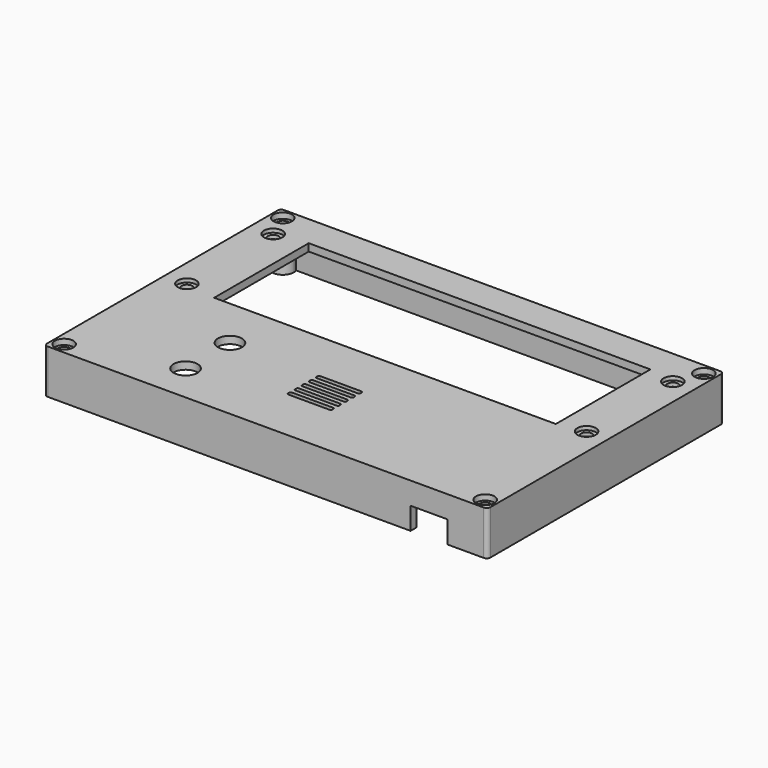
from build123d import *

# Parameters (mm, degrees)
F0_W            = 120
F0_H            = 80
F1_DEPTH        = 2
F3_DEPTH        = 12
F5_D            = 3
F5_CBORE_D      = 5
F5_CBORE_DEPTH  = 1
F4_W            = 92.5
F4_H            = 32
F6_DEPTH        = 3
F7_W            = 10
F7_H            = 6
F8_DEPTH        = 3
F9_R            = 1
F10_R           = 3.25
F11_DEPTH       = 2
F12_R           = 1.25
F13_DEPTH       = 1
F15_D           = 3.2
F15_CBORE_D     = 5
F15_CBORE_DEPTH = 1.5


# Not quite as in the source:
# - a feature names something its author has since deleted; it is built from what else it names


with BuildPart() as f1:
    # F0 (on Top) → F1 (new body)
    with BuildSketch(Plane.XY):
        Rectangle(F0_W, F0_H)
    extrude(amount=F1_DEPTH)

    # F2 (on face) → F3 (join)
    with BuildSketch(Plane.XY.offset(2)):
        with BuildLine():
            Line((-58, 38), (-54.1715728753, 38))
            ThreePointArc((-54.1715728753, 38), (-55.2679491924, 39.4494897428), (-57, 40))
            ThreePointArc((-57, 40), (-59.1213203436, 39.1213203436), (-60, 37))
            ThreePointArc((-60, 37), (-59.4494897428, 35.2679491924), (-58, 34.1715728753))
            Line((-58, 34.1715728753), (-58, 38))
        make_face()
        with BuildLine():
            ThreePointArc((-60, 37), (-59.1213203436, 39.1213203436), (-57, 40))
            Line((-57, 40), (-60, 40))
            Line((-60, 40), (-60, 37))
        make_face()
        with BuildLine():
            ThreePointArc((-54, 37), (-54.043204321, 37.5073059362), (-54.1715728753, 38))
            Line((-54.1715728753, 38), (-58, 38))
            Line((-58, 38), (-58, 34.1715728753))
            ThreePointArc((-58, 34.1715728753), (-55.2679491924, 34.5505102572), (-54, 37))
        make_face()
        with BuildLine():
            Line((-58, -34.1715728753), (-58, 34.1715728753))
            ThreePointArc((-58, 34.1715728753), (-59.4494897428, 35.2679491924), (-60, 37))
            Line((-60, 37), (-60, -37))
            ThreePointArc((-60, -37), (-59.4494897428, -35.2679491924), (-58, -34.1715728753))
        make_face()
        with BuildLine():
            Line((-54.1715728753, 38), (54.1715728753, 38))
            ThreePointArc((54.1715728753, 38), (55.2679491924, 39.4494897428), (57, 40))
            Line((57, 40), (-57, 40))
            ThreePointArc((-57, 40), (-55.2679491924, 39.4494897428), (-54.1715728753, 38))
        make_face()
        with BuildLine():
            Line((54.1715728753, 38), (58, 38))
            Line((58, 38), (58, 34.1715728753))
            ThreePointArc((58, 34.1715728753), (59.4494897428, 35.2679491924), (60, 37))
            ThreePointArc((60, 37), (59.1213203436, 39.1213203436), (57, 40))
            ThreePointArc((57, 40), (55.2679491924, 39.4494897428), (54.1715728753, 38))
        make_face()
        with BuildLine():
            Line((58, 34.1715728753), (58, 38))
            Line((58, 38), (54.1715728753, 38))
            ThreePointArc((54.1715728753, 38), (54.8786796564, 34.8786796564), (58, 34.1715728753))
        make_face()
        with BuildLine():
            Line((60, 40), (57, 40))
            ThreePointArc((57, 40), (59.1213203436, 39.1213203436), (60, 37))
            Line((60, 37), (60, 40))
        make_face()
        with BuildLine():
            ThreePointArc((60, 37), (59.4494897428, 35.2679491924), (58, 34.1715728753))
            Line((58, 34.1715728753), (58, -34.1715728753))
            ThreePointArc((58, -34.1715728753), (59.4494897428, -35.2679491924), (60, -37))
            Line((60, -37), (60, 37))
        make_face()
        with BuildLine():
            Line((60, -40), (60, -37))
            ThreePointArc((60, -37), (59.1213203436, -39.1213203436), (57, -40))
            Line((57, -40), (60, -40))
        make_face()
        with BuildLine():
            ThreePointArc((60, -37), (59.4494897428, -35.2679491924), (58, -34.1715728753))
            Line((58, -34.1715728753), (58, -38))
            Line((58, -38), (54.1715728753, -38))
            ThreePointArc((54.1715728753, -38), (55.2679491924, -39.4494897428), (57, -40))
            ThreePointArc((57, -40), (59.1213203436, -39.1213203436), (60, -37))
        make_face()
        with BuildLine():
            Line((58, -38), (58, -34.1715728753))
            ThreePointArc((58, -34.1715728753), (54.8786796564, -34.8786796564), (54.1715728753, -38))
            Line((54.1715728753, -38), (58, -38))
        make_face()
        with BuildLine():
            ThreePointArc((57, -40), (55.2679491924, -39.4494897428), (54.1715728753, -38))
            Line((54.1715728753, -38), (-54.1715728753, -38))
            ThreePointArc((-54.1715728753, -38), (-55.2679491924, -39.4494897428), (-57, -40))
            Line((-57, -40), (57, -40))
        make_face()
        with BuildLine():
            ThreePointArc((-57, -40), (-59.1213203436, -39.1213203436), (-60, -37))
            Line((-60, -37), (-60, -40))
            Line((-60, -40), (-57, -40))
        make_face()
        with BuildLine():
            ThreePointArc((-57, -40), (-55.2679491924, -39.4494897428), (-54.1715728753, -38))
            Line((-54.1715728753, -38), (-58, -38))
            Line((-58, -38), (-58, -34.1715728753))
            ThreePointArc((-58, -34.1715728753), (-59.4494897428, -35.2679491924), (-60, -37))
            ThreePointArc((-60, -37), (-59.1213203436, -39.1213203436), (-57, -40))
        make_face()
        with BuildLine():
            Line((-58, -38), (-54.1715728753, -38))
            ThreePointArc((-54.1715728753, -38), (-54.043204321, -37.5073059362), (-54, -37))
            ThreePointArc((-54, -37), (-55.2679491924, -34.5505102572), (-58, -34.1715728753))
            Line((-58, -34.1715728753), (-58, -38))
        make_face()
    extrude(amount=-F3_DEPTH)

    # F5 (through all)
    with Locations(Plane.XY.offset(2)):
        with Locations((-54, 30), (-54, 0.8), (54.2, 0.8), (54.2, 30)):
            CounterBoreHole(F5_D / 2, F5_CBORE_D / 2, F5_CBORE_DEPTH)

    # F4 (on face) → F6 (cut)
    with BuildSketch(Plane.XY.offset(2)):
        with Locations((0.75, 15.4)):
            Rectangle(F4_W, F4_H)
    extrude(amount=-F6_DEPTH, mode=Mode.SUBTRACT)

    # F7 (on face) → F8 (cut)
    with BuildSketch(Plane.XZ.offset(40)):
        with Locations((44.2, -7)):
            Rectangle(F7_W, F7_H)
    extrude(amount=-F8_DEPTH, mode=Mode.SUBTRACT)

    # F9
    f9_edges = [f1.edges().sort_by_distance(p)[0] for p in [
        (60, -40, -4),
        (60, 40, -4),
        (-60, -40, -4),
        (-60, 40, -4),
    ]]
    fillet(f9_edges, radius=F9_R)

    # F10 (on face) → F11 (cut, through all)
    with BuildSketch(Plane.XY.offset(2)):
        with Locations((-30, -14.6378241479)):
            Circle(F10_R)
        with Locations((-30, -29.6378241479)):
            Circle(F10_R)
        with BuildLine():
            Line((-5.6, -15.8000669783), (5.6, -15.8000669783))
            ThreePointArc((5.6, -15.8000669783), (5.8828427125, -15.6829096908), (6, -15.4000669783))
            Line((6, -15.4000669783), (6, -15.0000669783))
            ThreePointArc((6, -15.0000669783), (5.8828427125, -14.7172242658), (5.6, -14.6000669783))
            Line((5.6, -14.6000669783), (-5.6, -14.6000669783))
            ThreePointArc((-5.6, -14.6000669783), (-5.8828427125, -14.7172242658), (-6, -15.0000669783))
            Line((-6, -15.0000669783), (-6, -15.4000669783))
            ThreePointArc((-6, -15.4000669783), (-5.8828427125, -15.6829096908), (-5.6, -15.8000669783))
        make_face()
        with BuildLine():
            ThreePointArc((6, -17.4000669783), (5.8828427125, -17.1172242658), (5.6, -17.0000669783))
            Line((5.6, -17.0000669783), (-5.6, -17.0000669783))
            ThreePointArc((-5.6, -17.0000669783), (-5.8828427125, -17.1172242658), (-6, -17.4000669783))
            Line((-6, -17.4000669783), (-6, -17.8000669783))
            ThreePointArc((-6, -17.8000669783), (-5.8828427125, -18.0829096908), (-5.6, -18.2000669783))
            Line((-5.6, -18.2000669783), (5.6, -18.2000669783))
            ThreePointArc((5.6, -18.2000669783), (5.8828427125, -18.0829096908), (6, -17.8000669783))
            Line((6, -17.8000669783), (6, -17.4000669783))
        make_face()
        with BuildLine():
            ThreePointArc((6, -19.8000669783), (5.8828427125, -19.5172242658), (5.6, -19.4000669783))
            Line((5.6, -19.4000669783), (-5.6, -19.4000669783))
            ThreePointArc((-5.6, -19.4000669783), (-5.8828427125, -19.5172242658), (-6, -19.8000669783))
            Line((-6, -19.8000669783), (-6, -20.2000669783))
            ThreePointArc((-6, -20.2000669783), (-5.8828427125, -20.4829096908), (-5.6, -20.6000669783))
            Line((-5.6, -20.6000669783), (5.6, -20.6000669783))
            ThreePointArc((5.6, -20.6000669783), (5.8828427125, -20.4829096908), (6, -20.2000669783))
            Line((6, -20.2000669783), (6, -19.8000669783))
        make_face()
        with BuildLine():
            ThreePointArc((6, -22.2000669783), (5.8828427125, -21.9172242658), (5.6, -21.8000669783))
            Line((5.6, -21.8000669783), (-5.6, -21.8000669783))
            ThreePointArc((-5.6, -21.8000669783), (-5.8828427125, -21.9172242658), (-6, -22.2000669783))
            Line((-6, -22.2000669783), (-6, -22.6000669783))
            ThreePointArc((-6, -22.6000669783), (-5.8828427125, -22.8829096908), (-5.6, -23.0000669783))
            Line((-5.6, -23.0000669783), (5.6, -23.0000669783))
            ThreePointArc((5.6, -23.0000669783), (5.8828427125, -22.8829096908), (6, -22.6000669783))
            Line((6, -22.6000669783), (6, -22.2000669783))
        make_face()
        with BuildLine():
            ThreePointArc((6, -24.6000669783), (5.8828427125, -24.3172242658), (5.6, -24.2000669783))
            Line((5.6, -24.2000669783), (-5.6, -24.2000669783))
            ThreePointArc((-5.6, -24.2000669783), (-5.8828427125, -24.3172242658), (-6, -24.6000669783))
            Line((-6, -24.6000669783), (-6, -25.0000669783))
            ThreePointArc((-6, -25.0000669783), (-5.8828427125, -25.2829096908), (-5.6, -25.4000669783))
            Line((-5.6, -25.4000669783), (5.6, -25.4000669783))
            ThreePointArc((5.6, -25.4000669783), (5.8828427125, -25.2829096908), (6, -25.0000669783))
            Line((6, -25.0000669783), (6, -24.6000669783))
        make_face()
    extrude(amount=-F11_DEPTH, mode=Mode.SUBTRACT)

    # F12 (on face) → F13 (cut)
    with BuildSketch(Plane(origin=(0, 0, 0), x_dir=(1, 0, 0), z_dir=(0, 0, -1))):
        with Locations((17.5, 20.0000669783)):
            Circle(F12_R)
        with Locations((-17.5, 20.0000669783)):
            Circle(F12_R)
    extrude(amount=-F13_DEPTH, mode=Mode.SUBTRACT)

    # F15 (through all)
    with Locations(Plane.XY.offset(2)):
        with Locations((-57, 37), (57, 37), (57, -37), (-57, -37)):
            CounterBoreHole(F15_D / 2, F15_CBORE_D / 2, F15_CBORE_DEPTH)


solid = f1.part
